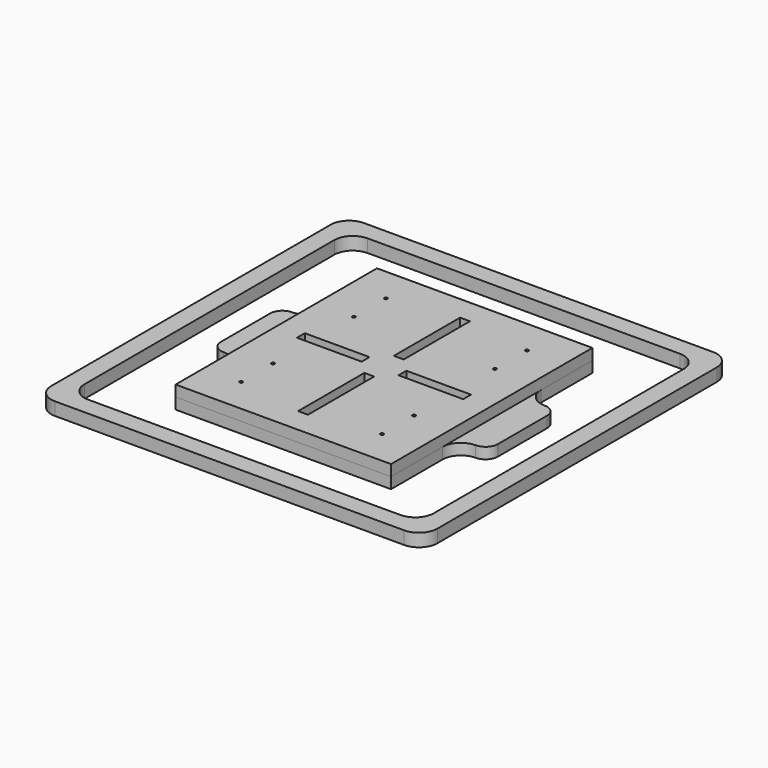
from build123d import *

# Parameters (mm, degrees)
F0_W              = 628
F0_H              = 628
F0_W_2            = 568
F0_H_2            = 568
F1_DEPTH          = 21
F2_R              = 30
F3_R              = 30
F4_W              = 61
F4_H              = 120
F5_DEPTH          = 18
F6_W              = 71
F6_H              = 137
F6_W_2            = 61
F6_H_2            = 120
F7_DEPTH          = 18.001
F7_COPIES2_COUNT  = 2
F7_COPIES2_PITCH  = 324.32631
F8_W              = 350.3333333333
F8_H              = 409.3333333333
F8_W_2            = 16
F8_H_2            = 134.6666666667
F8_W_3            = 105.1666666667
F8_H_3            = 16
F9_DEPTH          = 18
F10_R             = 2.5
F11_DEPTH         = 36.001
F11_COPIES2_COUNT = 2
F11_COPIES2_PITCH = 324.32631


# Not quite as in the source:
# - a pattern or mirror of a feature is missing from the dataset's text; its kind, count and spacing are read off the source's solid


with BuildPart() as f1:
    # F0 (on Top) → F1 (new body)
    with BuildSketch(Plane.XY):
        Rectangle(F0_W, F0_H)
        Rectangle(F0_W_2, F0_H_2, mode=Mode.SUBTRACT)
    extrude(amount=F1_DEPTH)

    # F2
    f2_edges = [f1.edges().sort_by_distance(p)[0] for p in [
        (-284, 284, 10.5),
        (284, 284, 10.5),
        (284, -284, 10.5),
        (-284, -284, 10.5),
    ]]
    fillet(f2_edges, radius=F2_R)

    # F3
    f3_edges = [f1.edges().sort_by_distance(p)[0] for p in [
        (-314, -314, 10.5),
        (314, -314, 10.5),
        (314, 314, 10.5),
        (-314, 314, 10.5),
    ]]
    fillet(f3_edges, radius=F3_R)


with BuildPart() as f5:
    # F4 (on Top) → F5 (new body)
    with BuildSketch(Plane.XY):
        with BuildLine():
            Line((-175.1666666667, -204.6666666667), (175.1666666667, -204.6666666667))
            Line((175.1666666667, -204.6666666667), (175.1666666667, -100))
            ThreePointArc((175.1666666667, -100), (183.9534632311, -78.7867965644), (205.1666666667, -70))
            ThreePointArc((205.1666666667, -70), (219.3088022904, -64.1421356237), (225.1666666667, -50))
            Line((225.1666666667, -50), (225.1666666667, 0))
            Line((225.1666666667, 0), (225.1666666667, 50))
            ThreePointArc((225.1666666667, 50), (219.3088022904, 64.1421356237), (205.1666666667, 70))
            ThreePointArc((205.1666666667, 70), (183.9534632311, 78.7867965644), (175.1666666667, 100))
            Line((175.1666666667, 100), (175.1666666667, 204.6666666667))
            Line((175.1666666667, 204.6666666667), (-175.1666666667, 204.6666666667))
            Line((-175.1666666667, 204.6666666667), (-175.1666666667, 100))
            ThreePointArc((-175.1666666667, 100), (-183.9534632311, 78.7867965644), (-205.1666666667, 70))
            ThreePointArc((-205.1666666667, 70), (-219.3088022904, 64.1421356237), (-225.1666666667, 50))
            Line((-225.1666666667, 50), (-225.1666666667, 0))
            Line((-225.1666666667, 0), (-225.1666666667, -50))
            ThreePointArc((-225.1666666667, -50), (-219.3088022904, -64.1421356237), (-205.1666666667, -70))
            ThreePointArc((-205.1666666667, -70), (-183.9534632311, -78.7867965644), (-175.1666666667, -100))
            Line((-175.1666666667, -100), (-175.1666666667, -204.6666666667))
        make_face()
        Polygon((-145.1666666667, -54.6666666667), (-114.6666666667, -54.6666666667), (-84.1666666667, -54.6666666667), (-84.1666666667, -174.6666666667), (-145.1666666667, -174.6666666667), align=None, mode=Mode.SUBTRACT)
        with Locations((114.6666666667, -114.6666666667)):
            Rectangle(F4_W, F4_H, mode=Mode.SUBTRACT)
        Polygon((-84.1666666667, 174.6666666667), (-84.1666666667, 54.6666666667), (-114.6666666667, 54.6666666667), (-145.1666666667, 54.6666666667), (-145.1666666667, 174.6666666667), align=None, mode=Mode.SUBTRACT)
        with Locations((114.6666666667, 114.6666666667)):
            Rectangle(F4_W, F4_H, mode=Mode.SUBTRACT)
    extrude(amount=F5_DEPTH)

    # F6 (on face) → F7 (cut, through all)
    with BuildSketch(Plane.XY.offset(18)):
        with Locations((-114.6666666667, 114.6666666667)):
            Rectangle(F6_W, F6_H)
        with Locations((-114.6666666667, 114.6666666667)):
            Rectangle(F6_W_2, F6_H_2, mode=Mode.SUBTRACT)
    f7 = extrude(amount=-F7_DEPTH, mode=Mode.SUBTRACT)

    # F7_copies: F7 across plane
    add(f7.mirror(Plane(origin=(0, 0, 0), x_dir=(0, 0, -1), z_dir=(0, -1, 0))), mode=Mode.SUBTRACT)

    # F7_copies1: F7 across plane
    add(f7.mirror(Plane(origin=(0, 0, 0), x_dir=(0, 0, 1), z_dir=(1, 0, 0))), mode=Mode.SUBTRACT)

    # F7_copies2: F7 ×2
    with Locations(*[Vector(0.7071067812, -0.7071067812, 0) * (i * F7_COPIES2_PITCH) for i in range(1, F7_COPIES2_COUNT)]):
        add(f7, mode=Mode.SUBTRACT)


with BuildPart() as f9:
    # F8 (on face) → F9 (new body)
    with BuildSketch(Plane.XY.offset(18)):
        Rectangle(F8_W, F8_H)
        with Locations((0, -97.3333333333)):
            Rectangle(F8_W_2, F8_H_2, mode=Mode.SUBTRACT)
        with Locations((-82.5833333333, 0)):
            Rectangle(F8_W_3, F8_H_3, mode=Mode.SUBTRACT)
        with Locations((0, 97.3333333333)):
            Rectangle(F8_W_2, F8_H_2, mode=Mode.SUBTRACT)
        with Locations((82.5833333333, 0)):
            Rectangle(F8_W_3, F8_H_3, mode=Mode.SUBTRACT)
    extrude(amount=F9_DEPTH)

    # F10 (on face) → F11 (cut, through all)
    with BuildSketch(Plane.XY.offset(36)):
        with Locations((-114.6666666667, 147.1666666667)):
            Circle(F10_R)
        with Locations((-114.6666666667, 82.1666666667)):
            Circle(F10_R)
    f11 = extrude(amount=-F11_DEPTH, mode=Mode.SUBTRACT)

    # F11_copies: F11 across plane
    add(f11.mirror(Plane(origin=(0, 0, 0), x_dir=(0, 0, 1), z_dir=(1, 0, 0))), mode=Mode.SUBTRACT)

    # F11_copies1: F11 across plane
    add(f11.mirror(Plane(origin=(0, 0, 0), x_dir=(0, 0, -1), z_dir=(0, -1, 0))), mode=Mode.SUBTRACT)

    # F11_copies2: F11 ×2
    with Locations(*[Vector(0.7071067812, -0.7071067812, 0) * (i * F11_COPIES2_PITCH) for i in range(1, F11_COPIES2_COUNT)]):
        add(f11, mode=Mode.SUBTRACT)


solid = Compound([f1.part, f5.part, f9.part])
